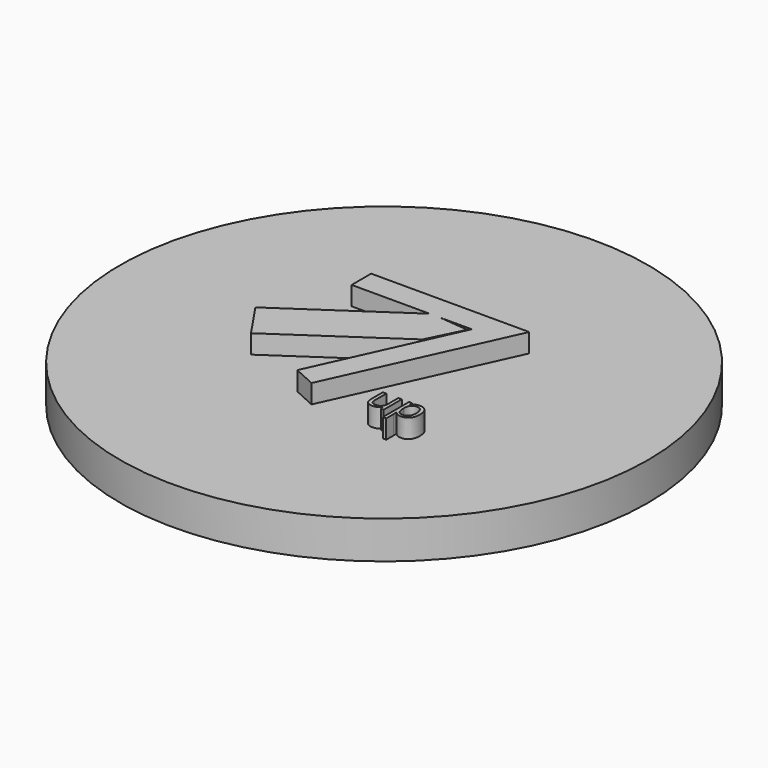
from build123d import *

# Parameters (mm, degrees)
F0_R         = 44.45
F1_DEPTH     = 6.35
F4_DEPTH     = 3.175
F7_TEXT_SIZE = 7.1167971732
F8_DEPTH     = 3.175


# Not quite as in the source:
# - the program builds the solid bodies; features that only make, move or delete a surface that nothing else refers to are left out
# - Text() gives the source's letters only with a copy of the font that has no kerning and outlines rounded to 1/6400 em; it was checked with that copy


with BuildPart() as f1:
    # F0 (on Top) → F1 (new body)
    with BuildSketch(Plane.XY):
        Circle(F0_R)
    extrude(amount=F1_DEPTH)

    # F2 (on face) + F3 (on face) → F4 (join)
    with BuildSketch(Plane.XY.offset(6.35)):
        Polygon((13.2779348642, 13.9486901462), (-13.3322151378, 13.9486901462), (-13.3322151378, 9.8365536903), (6.8819859699, 9.8365536903), (-3.7532192844, -13.5737807454), (0, -15.2788506821), align=None)
    with BuildSketch(Plane.XY.offset(6.35)):
        Polygon((0, 9.9786977635), (-19.2213449627, -3.0643560458), (-15.0771420449, -9.1716032475), (3.6446399161, 3.5324614262), (6.51634112, 9.3682538718), align=None)
    extrude(amount=F4_DEPTH)

    # F7 (on face) → F8 (join)
    with BuildSketch(Plane.XY.offset(6.35)):
        with Locations((8.4037585184, -15.2848567814)):
            Text('up', F7_TEXT_SIZE, font='Open Sans', text_align=(TextAlign.LEFT, TextAlign.BOTTOM))
    extrude(amount=F8_DEPTH)


solid = f1.part
